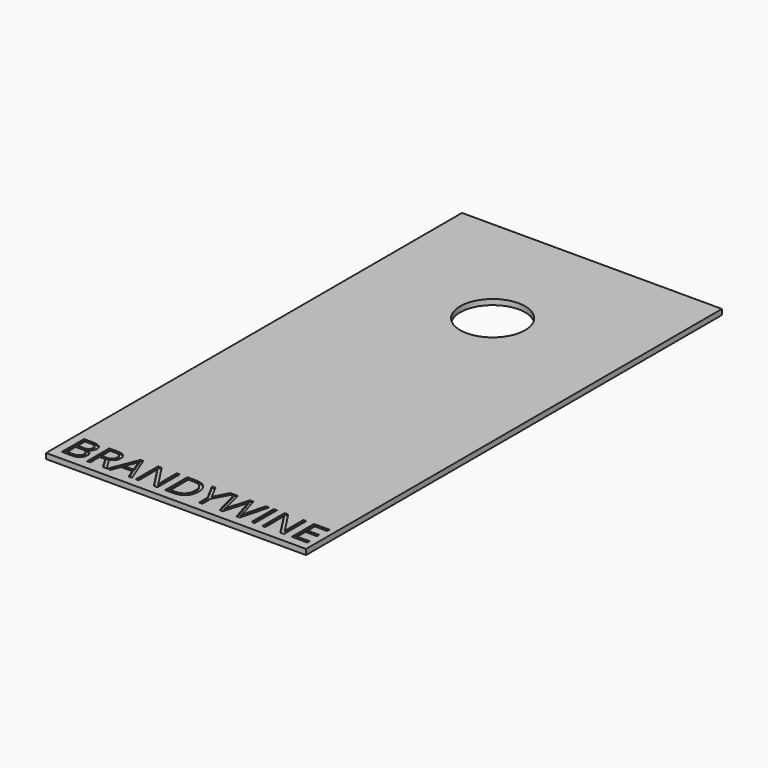
from build123d import *

# Parameters (mm, degrees)
F0_W         = 609.6
F0_H         = 1219.2
F0_R         = 76.2
F1_DEPTH     = 12.7
F2_TEXT_SIZE = 91.3723268443
F3_DEPTH     = 3.175


# Not quite as in the source:
# - Text() gives the source's letters only with a copy of the font that has no kerning and outlines rounded to 1/6400 em; it was checked with that copy


with BuildPart() as f1:
    # F0 (on Top) → F1 (new body)
    with BuildSketch(Plane.XY):
        with Locations((245.1588064432, 629.1477186379)):
            Rectangle(F0_W, F0_H)
        with Locations((245.1588064432, 947.6883411407)):
            Circle(F0_R, mode=Mode.SUBTRACT)
    extrude(amount=F1_DEPTH)

    # F2 (on face) → F3 (cut)
    with BuildSketch(Plane.XY.offset(12.7)):
        with Locations((-48.7719401717, 40.8194735646)):
            Text('BRANDYWINE', F2_TEXT_SIZE, font='Open Sans', text_align=(TextAlign.LEFT, TextAlign.BOTTOM))
    extrude(amount=-F3_DEPTH, mode=Mode.SUBTRACT)


solid = f1.part
